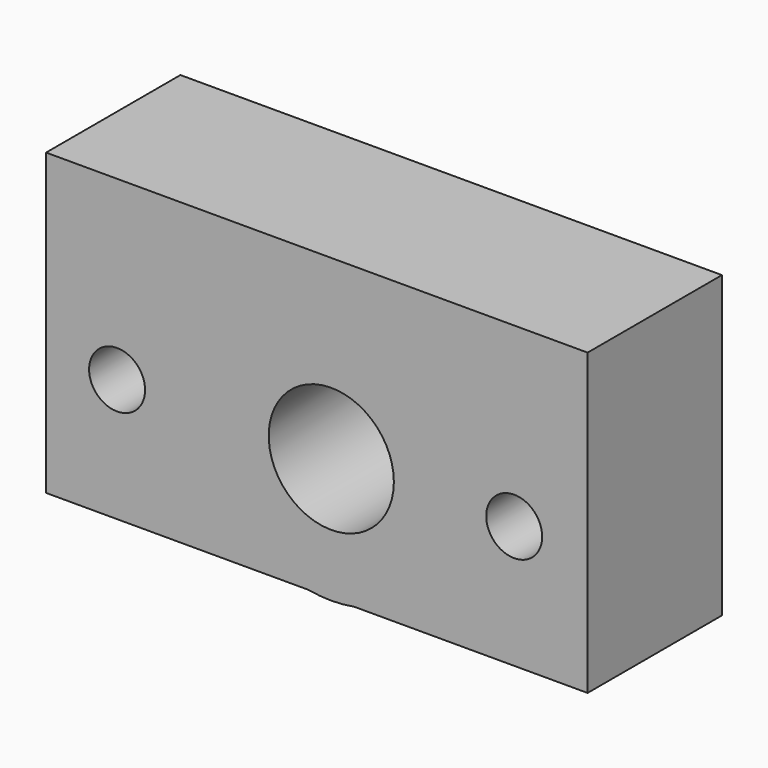
from build123d import *

# Parameters (mm, degrees)
F0_R     = 14.1997272149
F0_R_2   = 6.35
F2_DEPTH = 12.7
F3_DEPTH = 25.4


# Not quite as in the source:
# - the program builds the solid bodies; features that only make, move or delete a surface that nothing else refers to are left out


with BuildPart() as f2:
    # F0 (on Front) → F2 (new body)
    with BuildSketch(Plane.XZ):
        with BuildLine():
            ThreePointArc((5.1667592351, -27.8533101082), (21.7815136707, -18.1126460571), (28.3284712785, 0))
            ThreePointArc((28.3284712785, 0), (-18.1126460571, 21.7815136707), (-5.1667592351, -27.8533101082))
            Line((-5.1667592351, -27.8533101082), (5.1667592351, -27.8533101082))
        make_face()
        Circle(F0_R, mode=Mode.SUBTRACT)
        with BuildLine():
            ThreePointArc((-5.1667592351, -27.8533101082), (-18.1126460571, 21.7815136707), (28.3284712785, 0))
            ThreePointArc((28.3284712785, 0), (21.7815136707, -18.1126460571), (5.1667592351, -27.8533101082))
            Line((5.1667592351, -27.8533101082), (58.1642687321, -27.8533101082))
            Line((58.1642687321, -27.8533101082), (58.1642687321, 40.1415377855))
            Line((58.1642687321, 40.1415377855), (-64.7179856896, 40.1415377855))
            Line((-64.7179856896, 40.1415377855), (-64.7179856896, -27.8533101082))
            Line((-64.7179856896, -27.8533101082), (-5.1667592351, -27.8533101082))
        make_face()
        with Locations((-48.6067570746, 0)):
            Circle(F0_R_2, mode=Mode.SUBTRACT)
        with Locations((41.5068976581, 0)):
            Circle(F0_R_2, mode=Mode.SUBTRACT)
        with BuildLine():
            Line((5.1667592351, -27.8533101082), (-5.1667592351, -27.8533101082))
            ThreePointArc((-5.1667592351, -27.8533101082), (0, -28.3284712785), (5.1667592351, -27.8533101082))
        make_face()
    extrude(amount=F2_DEPTH)

    # F3 (add): a face of the model
    f3_faces = [f2.faces().sort_by_distance(p)[0] for p in [
        (56.7575636957, -12.7, 6.1441138387),
    ]]
    extrude(f3_faces, amount=F3_DEPTH)


solid = f2.part
